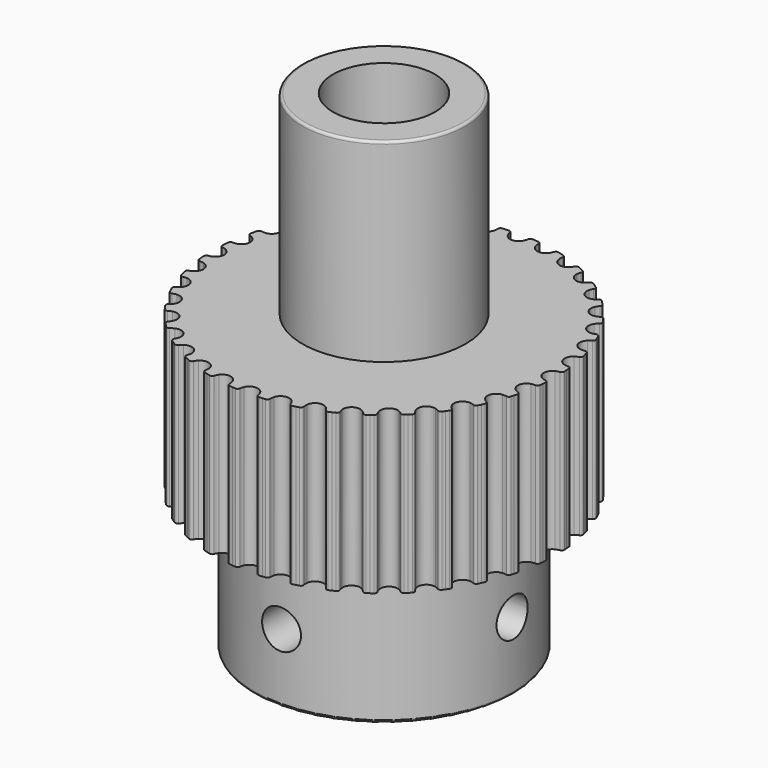
from build123d import *

# Parameters (mm, degrees)
F3_DEPTH  = 7.6962
F4_COUNT  = 36
F5_R      = 12.7
F6_DEPTH  = 13.335
F7_R      = 6.35
F8_DEPTH  = 1.143
F9_R      = 1.905
F10_DEPTH = 16.7695702545
F11_R     = 1.905
F12_DEPTH = 13
F13_R     = 8.001
F14_DEPTH = 19.05
F15_R     = 5
F16_DEPTH = 48.9214
F17_R     = 0.25


# Not quite as in the source:
# - a feature names something its author has since deleted; it is built from what else it names


with BuildPart() as f3:
    # F2 (on Top) → F3 (new body, symmetric)
    with BuildSketch(Plane.XY):
        with BuildLine():
            ThreePointArc((0.7737107197, 16.1672889306), (0.4600755233, 15.8045189969), (0, 15.6692430785))
            ThreePointArc((0, 15.6692430785), (-0.4600755233, 15.8045189969), (-0.7737107197, 16.1672889306))
            ThreePointArc((-0.7737107197, 16.1672889306), (-0.8456427107, 16.3586085585), (-0.8912557136, 16.5578492807))
            ThreePointArc((-0.8912557136, 16.5578492807), (-0.9824897662, 16.7141965786), (-1.1553353273, 16.7679789356))
            ThreePointArc((-1.1553353273, 16.7679789356), (-1.3101688198, 16.7565919855), (-1.4648905279, 16.7437753522))
            Line((-1.4648905279, 16.7437753522), (0, 0))
            Line((0, 0), (1.4648905279, 16.7437753522))
            ThreePointArc((1.4648905279, 16.7437753522), (1.3101688198, 16.7565919855), (1.1553353273, 16.7679789356))
            ThreePointArc((1.1553353273, 16.7679789356), (0.9824897662, 16.7141965786), (0.8912557136, 16.5578492807))
            ThreePointArc((0.8912557136, 16.5578492807), (0.8456427107, 16.3586085585), (0.7737107197, 16.1672889306))
        make_face()
    extrude(amount=F3_DEPTH, both=True)

    # F4: F3 ×36 about axis
    f4_axis = Axis((0, 0, 0), (0, 0, -1))


with BuildPart() as f3_1:
    add(f3.part)
    for i in range(1, F4_COUNT):
        add(f3.part.rotate(f4_axis, i * 360 / F4_COUNT))

    # F5 (on face) → F6 (join)
    with BuildSketch(Plane(origin=(0, 0, -7.6962), x_dir=(1, 0, 0), z_dir=(0, 0, -1))):
        Circle(F5_R)
    extrude(amount=F6_DEPTH)

    # F7 (on face) → F8 (join)
    with BuildSketch(Plane(origin=(0, 0, -21.0312), x_dir=(1, 0, 0), z_dir=(0, 0, -1))):
        Circle(F7_R)
    extrude(amount=F8_DEPTH)

    # F9 (on Front) → F10 (cut, through all)
    with BuildSketch(Plane.XZ):
        with Locations((0, -14.3637)):
            Circle(F9_R)
    extrude(amount=F10_DEPTH, mode=Mode.SUBTRACT)

    # F11 (on Right) → F12 (cut, symmetric)
    with BuildSketch(Plane.YZ):
        with Locations((0, -14.3637)):
            Circle(F11_R)
    extrude(amount=F12_DEPTH, both=True, mode=Mode.SUBTRACT)

    # F13 (on face) → F14 (join)
    with BuildSketch(Plane.XY.offset(7.6962)):
        Circle(F13_R)
    extrude(amount=F14_DEPTH)

    # F15 (on face) → F16 (cut, through all)
    with BuildSketch(Plane.XY.offset(26.7462)):
        Circle(F15_R)
    extrude(amount=-F16_DEPTH, mode=Mode.SUBTRACT)

    # F17
    f17_edges = [f3_1.edges().sort_by_distance(p)[0] for p in [
        (-12.7, 0, -21.0312),
        (-8.001, 0, 26.7462),
    ]]
    fillet(f17_edges, radius=F17_R)


solid = f3_1.part
